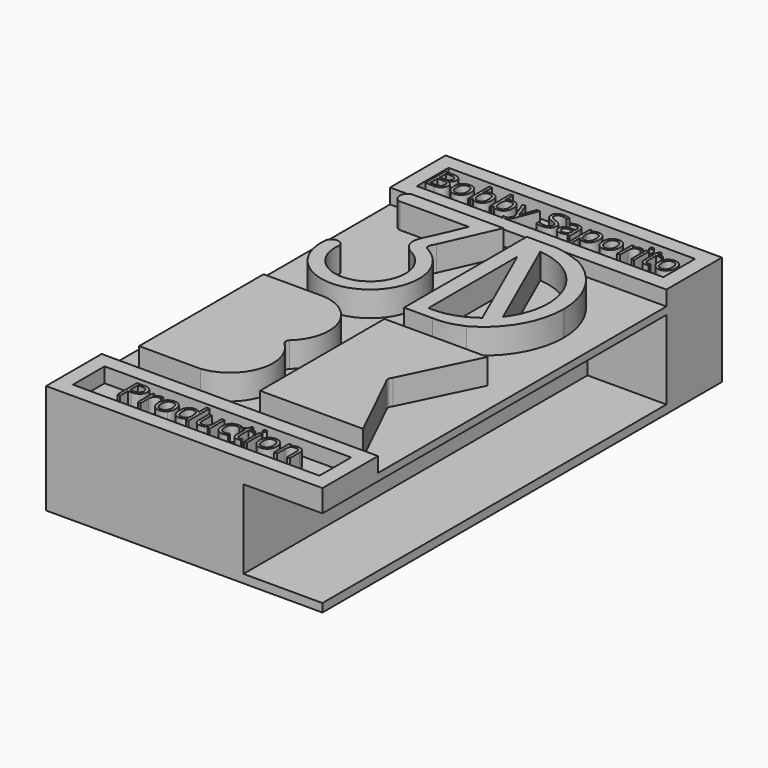
from build123d import *

# Parameters (mm, degrees)
F1_W           = 55.6107703596
F1_H           = 92.8997322917
F2_DEPTH       = 19.05
F3_DEPTH       = 5.08
F5_DEPTH       = 3
F6_DEPTH       = 3
F7_W           = 55.6107703596
F7_H           = 3.7946861994
F8_DEPTH       = 19.05
F9_W           = 55.6107703596
F9_H           = 3.7949544203
F10_DEPTH      = 19.05
F11_W          = 15.875
F11_H          = 7.9375
F11_W_2        = 15.8749995753
F12_DEPTH      = 86.5193729115
F4_TEXT_SIZE   = 6.9556654327
F13_DEPTH      = 3
F4_TEXT_SIZE_2 = 6.995924438
F14_DEPTH      = 3


# Not quite as in the source:
# - ends of sketch curves that miss each other by under 0.0002 mm in the source are joined
# - a feature names something its author has since deleted; it is built from what else it names
# - Text() gives the source's letters only with a copy of the font that has no kerning and outlines rounded to 1/6400 em; it was checked with that copy


with BuildPart() as f2:
    # F1 (on Top) → F2 (new body)
    with BuildSketch(Plane.XY):
        with Locations((-0.0001015142, 0.0001341105)):
            Rectangle(F1_W, F1_H)
    extrude(amount=-F2_DEPTH)

    # F0 (on Top) → F3 (join)
    with BuildSketch(Plane.XY):
        with BuildLine():
            Line((1.9535701722, 33.4806852043), (1.9535701722, 2.6171170175))
            Line((1.9535701722, 2.6171170175), (7.6673883013, 2.6171170175))
            add(Edge.make_bspline(
                [(13.5640528841, 3.8033656441), (12.5585792201, 3.4051600509), (10.5947152477, 2.6273956539), (8.6274422547, 2.6204880265), (7.6673883013, 2.6171170175)],
                knots=[0, 0, 0, 0, 0.5119874279, 1, 1, 1, 1], degree=3))
            ThreePointArc((13.5640528841, 3.8033656441), (19.5771167094, 9.6257290209), (21.8482203782, 17.6817168551))
            Line((21.8482203782, 17.6817168551), (21.8482203782, 18.0489011109))
            ThreePointArc((21.8482203782, 18.0489011109), (19.5771167094, 26.1048889451), (13.5640528841, 31.9272523219))
            add(Edge.make_bspline(
                [(13.5640528841, 31.9272523219), (12.0188625137, 32.4806988664), (9.5071250594, 33.3803371514), (8.1786150797, 33.4528004476), (7.6673883013, 33.4806852043)],
                knots=[0, 0, 0, 0, 0.6151878524, 1, 1, 1, 1], degree=3))
            Line((7.6673883013, 33.4806852043), (1.9535701722, 33.4806852043))
        make_face()
        with BuildLine():
            ThreePointArc((13.7255926495, 7.5781230036), (9.6198125415, 5.4448354943), (5.0269701927, 4.8843490524))
            Line((5.0269701927, 4.8843490524), (5.0269701927, 27.2558980547))
            Line((5.0269701927, 27.2558980547), (13.7255926495, 7.5781230036))
        make_face(mode=Mode.SUBTRACT)
        with BuildLine():
            ThreePointArc((6.7811124511, 30.8286115181), (17.6657420253, 23.1223286699), (16.0391214303, 9.8854082672))
            Line((16.0391214303, 9.8854082672), (6.7811124511, 30.8286115181))
        make_face(mode=Mode.SUBTRACT)
        with BuildLine():
            Line((-7.5453622267, 22.6989928633), (-2.7351737954, 33.4806852043))
            Line((-2.7351737954, 33.4806852043), (-21.1572051048, 33.4806852043))
            ThreePointArc((-21.1572051048, 33.4806852043), (-22.3890896886, 31.9530339911), (-21.1572051048, 30.425382778))
            Line((-21.1572051048, 30.425382778), (-7.2931135073, 30.425382778))
            Line((-7.2931135073, 30.425382778), (-9.4495294616, 25.3879800439))
            add(Edge.make_bspline(
                [(-9.4495294616, 25.3879800439), (-10.3302159731, 23.6726618568), (-11.8808970013, 20.6523914937), (-10.1830913379, 19.0052173822), (-9.4495294616, 18.2935316116)],
                knots=[0, 0, 0, 0, 0.5679353107, 1, 1, 1, 1], degree=3))
            ThreePointArc((-9.4495294616, 18.2935316116), (-8.744805336, 5.5966861339), (-19.1914085299, 12.8475483507))
            ThreePointArc((-19.1914085299, 12.8475483507), (-20.5873309935, 13.9352987723), (-21.9832534571, 12.8475483507))
            ThreePointArc((-21.9832534571, 12.8475483507), (-7.5716745464, 3.0830422585), (-7.6246123494, 20.4909825018))
            add(Edge.make_bspline(
                [(-7.5453622267, 22.6989928633), (-7.8757345138, 22.1285959519), (-8.4306078493, 21.1705917574), (-7.8693930702, 20.681447967), (-7.6246123494, 20.4909825018)],
                knots=[0, 0, 0, 0, 0.5706142153, 0.9583691649, 0.9583691649, 0.9583691649, 0.9583691649], degree=3))
        make_face()
        with BuildLine():
            Line((1.9535701722, -33.6182080209), (21.8482203782, -33.6182080209))
            Line((21.8482203782, -33.6182080209), (22.670282051, -33.6182080209))
            Line((22.670282051, -33.6182080209), (15.4876355082, -18.8196848612))
            add(Edge.make_bspline(
                [(15.4876355082, -18.8196848612), (15.371168109, -18.6560732739), (15.159509665, -18.3587387901), (15.1679139181, -18.0863425739), (15.171693638, -17.9638353875)],
                knots=[0, 0, 0, 0, 0.550261057, 1, 1, 1, 1], degree=3))
            add(Edge.make_bspline(
                [(15.4876355082, -17.1079859138), (15.371168109, -17.2715975011), (15.159509665, -17.5689319849), (15.1679139181, -17.8413282011), (15.171693638, -17.9638353875)],
                knots=[0, 0, 0, 0, 0.550261057, 1, 1, 1, 1], degree=3))
            Line((15.4876355082, -17.1079859138), (22.670282051, -2.3094627541))
            Line((22.670282051, -2.3094627541), (1.9535701722, -2.3094627541))
            Line((1.9535701722, -2.3094627541), (1.9535701722, -33.6182080209))
        make_face()
        with BuildLine():
            Line((-22.3890896886, -2.3094627541), (-22.3890896886, -33.6182080209))
            Line((-22.3890896886, -33.6182080209), (-10.0687015802, -33.6182080209))
            ThreePointArc((-10.0687015802, -33.6182080209), (-2.7489802993, -27.706179837), (-5.1699676551, -18.6139184516))
            add(Edge.make_bspline(
                [(-5.1699676551, -18.6139184516), (-5.2577137292, -18.4897791328), (-5.4173213156, -18.2639732804), (-5.4122223799, -18.0570156997), (-5.4099266417, -17.9638353875)],
                knots=[0, 0, 0, 0, 0.5497612996, 1, 1, 1, 1], degree=3))
            add(Edge.make_bspline(
                [(-5.1699676551, -17.3137523234), (-5.2577137292, -17.4378916422), (-5.4173213156, -17.6636974946), (-5.4122223799, -17.8706550753), (-5.4099266417, -17.9638353875)],
                knots=[0, 0, 0, 0, 0.5497612996, 1, 1, 1, 1], degree=3))
            ThreePointArc((-5.1699676551, -17.3137523234), (-2.7489802993, -8.221490938), (-10.0687015802, -2.3094627541))
            Line((-10.0687015802, -2.3094627541), (-22.3890896886, -2.3094627541))
        make_face()
    extrude(amount=F3_DEPTH)

    # F4 (on face) → F5 (join)
    with BuildSketch(Plane.XY):
        Polygon((-27.805486694, 46.4500002563), (-27.805486694, 36.2746864557), (27.8052836657, 36.2746864557), (27.8052836657, 46.4500002563), (24.8052836657, 46.4500002563), (24.8052836657, 39.2746864557), (-24.805486694, 39.2746864557), (-24.805486694, 46.4500002563), align=None)
        Polygon((-27.805486694, 50.2446864557), (-27.805486694, 46.4500002563), (-24.805486694, 46.4500002563), (-24.805486694, 47.2446864557), (24.8052836657, 47.2446864557), (24.8052836657, 46.4500002563), (27.8052836657, 46.4500002563), (27.8052836657, 50.2446864557), align=None)
    extrude(amount=F5_DEPTH)

    # F4 (on face) → F6 (join)
    with BuildSketch(Plane.XY):
        Polygon((27.8052836657, -36.2746864557), (-27.805486694, -36.2746864557), (-27.805486694, -46.4497320354), (-24.805486694, -46.4497320354), (-24.805486694, -39.2746864557), (24.8052836657, -39.2746864557), (24.8052836657, -46.4497320354), (27.8052836657, -46.4497320354), align=None)
        Polygon((-24.805486694, -46.4497320354), (-27.805486694, -46.4497320354), (-27.805486694, -50.2446864557), (27.8052836657, -50.2446864557), (27.8052836657, -46.4497320354), (24.8052836657, -46.4497320354), (24.8052836657, -47.2446864557), (-24.805486694, -47.2446864557), align=None)
        with BuildLine():
            add(Edge.make_bspline(
                [(-14.0935817981, -41.9836251579), (-14.0935817981, -42.7422457142), (-14.6111708952, -43.1505234919)],
                knots=[0, 0, 0, 1, 1, 1], degree=2))
            add(Edge.make_bspline(
                [(-15.9649915853, -40.5286914975), (-14.0935817981, -40.5286914975), (-14.0935817981, -41.9836251579)],
                knots=[0, 0, 0, 1, 1, 1], degree=2))
            Line((-15.9649915853, -40.5286914975), (-17.2603307195, -40.5286914975))
            Line((-17.2603307195, -40.5286914975), (-17.2603307195, -45.5231256783))
            Line((-17.2603307195, -45.5231256783), (-16.6798876138, -45.5231256783))
            Line((-16.6798876138, -45.5231256783), (-16.6798876138, -43.5588012697))
            Line((-16.6798876138, -43.5588012697), (-16.0917927157, -43.5588012697))
            add(Edge.make_bspline(
                [(-14.6111708952, -43.1505234919), (-15.1287599923, -43.5588012697), (-16.0917927157, -43.5588012697)],
                knots=[0, 0, 0, 1, 1, 1], degree=2))
        make_face()
        with BuildLine():
            Line((-16.1562863941, -43.0603416535), (-16.6798876138, -43.0603416535))
            Line((-16.6798876138, -43.0603416535), (-16.6798876138, -41.0315235664))
            Line((-16.6798876138, -41.0315235664), (-16.0305783769, -41.0315235664))
            add(Edge.make_bspline(
                [(-15.0194486729, -41.2736481388), (-15.3441032914, -41.0315235664), (-16.0305783769, -41.0315235664)],
                knots=[0, 0, 0, 1, 1, 1], degree=2))
            add(Edge.make_bspline(
                [(-14.6947940545, -42.0109529878), (-14.6947940545, -41.5157727111), (-15.0194486729, -41.2736481388)],
                knots=[0, 0, 0, 1, 1, 1], degree=2))
            add(Edge.make_bspline(
                [(-15.039671267, -42.8111118454), (-14.6947940545, -42.5618820373), (-14.6947940545, -42.0109529878)],
                knots=[0, 0, 0, 1, 1, 1], degree=2))
            add(Edge.make_bspline(
                [(-16.1562863941, -43.0603416535), (-15.3845484795, -43.0603416535), (-15.039671267, -42.8111118454)],
                knots=[0, 0, 0, 1, 1, 1], degree=2))
        make_face(mode=Mode.SUBTRACT)
        with BuildLine():
            add(Edge.make_bspline(
                [(-7.0462810399, -43.6473434384), (-7.0462810399, -44.5633722945), (-7.507028251, -45.077682052)],
                knots=[0, 0, 0, 1, 1, 1], degree=2))
            add(Edge.make_bspline(
                [(-7.5092144774, -42.2334015226), (-7.0462810399, -42.7564561857), (-7.0462810399, -43.6473434384)],
                knots=[0, 0, 0, 1, 1, 1], degree=2))
            add(Edge.make_bspline(
                [(-8.7570031877, -41.7103468596), (-7.9721479148, -41.7103468596), (-7.5092144774, -42.2334015226)],
                knots=[0, 0, 0, 1, 1, 1], degree=2))
            add(Edge.make_bspline(
                [(-10.0282938317, -42.2213772775), (-9.5702794036, -41.7103468596), (-8.7570031877, -41.7103468596)],
                knots=[0, 0, 0, 1, 1, 1], degree=2))
            add(Edge.make_bspline(
                [(-10.4863082597, -43.6473434384), (-10.4863082597, -42.7324076954), (-10.0282938317, -42.2213772775)],
                knots=[0, 0, 0, 1, 1, 1], degree=2))
            add(Edge.make_bspline(
                [(-10.2742443002, -44.679242293), (-10.4863082597, -44.238717676), (-10.4863082597, -43.6473434384)],
                knots=[0, 0, 0, 1, 1, 1], degree=2))
            add(Edge.make_bspline(
                [(-9.6730320438, -45.3558793597), (-10.0621803407, -45.1197669099), (-10.2742443002, -44.679242293)],
                knots=[0, 0, 0, 1, 1, 1], degree=2))
            add(Edge.make_bspline(
                [(-8.7810516779, -45.5919918095), (-9.2838837469, -45.5919918095), (-9.6730320438, -45.3558793597)],
                knots=[0, 0, 0, 1, 1, 1], degree=2))
            add(Edge.make_bspline(
                [(-7.507028251, -45.077682052), (-7.967775462, -45.5919918095), (-8.7810516779, -45.5919918095)],
                knots=[0, 0, 0, 1, 1, 1], degree=2))
        make_face()
        with BuildLine():
            add(Edge.make_bspline(
                [(-9.8982133616, -43.6473434384), (-9.8982133616, -44.3655188064), (-9.6112711484, -44.7410031884)],
                knots=[0, 0, 0, 1, 1, 1], degree=2))
            add(Edge.make_bspline(
                [(-9.6145504879, -42.5580561411), (-9.8982133616, -42.9237025043), (-9.8982133616, -43.6473434384)],
                knots=[0, 0, 0, 1, 1, 1], degree=2))
            add(Edge.make_bspline(
                [(-8.7744929988, -42.1924097779), (-9.3308876142, -42.1924097779), (-9.6145504879, -42.5580561411)],
                knots=[0, 0, 0, 1, 1, 1], degree=2))
            add(Edge.make_bspline(
                [(-7.9218647079, -42.5629751505), (-8.210446591, -42.1924097779), (-8.7744929988, -42.1924097779)],
                knots=[0, 0, 0, 1, 1, 1], degree=2))
            add(Edge.make_bspline(
                [(-7.6332828248, -43.6473434384), (-7.6332828248, -42.933540523), (-7.9218647079, -42.5629751505)],
                knots=[0, 0, 0, 1, 1, 1], degree=2))
            add(Edge.make_bspline(
                [(-7.9218647079, -44.7426428582), (-7.6332828248, -44.368798146), (-7.6332828248, -43.6473434384)],
                knots=[0, 0, 0, 1, 1, 1], degree=2))
            add(Edge.make_bspline(
                [(-8.7679343196, -45.1164875703), (-8.210446591, -45.1164875703), (-7.9218647079, -44.7426428582)],
                knots=[0, 0, 0, 1, 1, 1], degree=2))
            add(Edge.make_bspline(
                [(-9.6112711484, -44.7410031884), (-9.3243289351, -45.1164875703), (-8.7679343196, -45.1164875703)],
                knots=[0, 0, 0, 1, 1, 1], degree=2))
        make_face(mode=Mode.SUBTRACT)
        with BuildLine():
            Line((-3.5341083494, -45.0213867225), (-3.50350118, -45.0213867225))
            Line((-3.50350118, -45.0213867225), (-3.4280763696, -45.5231256783))
            Line((-3.4280763696, -45.5231256783), (-2.966782602, -45.5231256783))
            Line((-2.966782602, -45.5231256783), (-2.966782602, -40.2073162186))
            Line((-2.966782602, -40.2073162186), (-3.5341083494, -40.2073162186))
            Line((-3.5341083494, -40.2073162186), (-3.5341083494, -41.7311160102))
            Line((-3.5341083494, -41.7311160102), (-3.5198978779, -41.9945562899))
            Line((-3.5198978779, -41.9945562899), (-3.4958493876, -42.2645552486))
            Line((-3.4958493876, -42.2645552486), (-3.5406670286, -42.2645552486))
            add(Edge.make_bspline(
                [(-4.7092050324, -41.7103468596), (-3.9473051365, -41.7103468596), (-3.5406670286, -42.2645552486)],
                knots=[0, 0, 0, 1, 1, 1], degree=2))
            add(Edge.make_bspline(
                [(-5.8504152063, -42.2230169473), (-5.4404977588, -41.7103468596), (-4.7092050324, -41.7103468596)],
                knots=[0, 0, 0, 1, 1, 1], degree=2))
            add(Edge.make_bspline(
                [(-6.2603326539, -43.6615539099), (-6.2603326539, -42.735687035), (-5.8504152063, -42.2230169473)],
                knots=[0, 0, 0, 1, 1, 1], degree=2))
            add(Edge.make_bspline(
                [(-5.8520548761, -45.0897062971), (-6.2603326539, -44.5874207847), (-6.2603326539, -43.6615539099)],
                knots=[0, 0, 0, 1, 1, 1], degree=2))
            add(Edge.make_bspline(
                [(-4.7092050324, -45.5919918095), (-5.4437770984, -45.5919918095), (-5.8520548761, -45.0897062971)],
                knots=[0, 0, 0, 1, 1, 1], degree=2))
            add(Edge.make_bspline(
                [(-3.5341083494, -45.0213867225), (-3.9265359859, -45.5919918095), (-4.7092050324, -45.5919918095)],
                knots=[0, 0, 0, 1, 1, 1], degree=2))
        make_face()
        with BuildLine():
            add(Edge.make_bspline(
                [(-4.6370595616, -45.1164875703), (-4.0566164559, -45.1164875703), (-3.7953624026, -44.8005778574)],
                knots=[0, 0, 0, 1, 1, 1], degree=2))
            add(Edge.make_bspline(
                [(-5.4093440328, -44.7508412071), (-5.1464503097, -45.1164875703), (-4.6370595616, -45.1164875703)],
                knots=[0, 0, 0, 1, 1, 1], degree=2))
            add(Edge.make_bspline(
                [(-5.6722377558, -43.668112589), (-5.6722377558, -44.3851948439), (-5.4093440328, -44.7508412071)],
                knots=[0, 0, 0, 1, 1, 1], degree=2))
            add(Edge.make_bspline(
                [(-5.407704363, -42.5733597258), (-5.6722377558, -42.9608683529), (-5.6722377558, -43.668112589)],
                knots=[0, 0, 0, 1, 1, 1], degree=2))
            add(Edge.make_bspline(
                [(-4.6436182408, -42.1858510987), (-5.1431709702, -42.1858510987), (-5.407704363, -42.5733597258)],
                knots=[0, 0, 0, 1, 1, 1], degree=2))
            add(Edge.make_bspline(
                [(-3.7986417422, -42.5258093019), (-4.063175135, -42.1858510987), (-4.6436182408, -42.1858510987)],
                knots=[0, 0, 0, 1, 1, 1], degree=2))
            add(Edge.make_bspline(
                [(-3.5341083494, -43.6615539099), (-3.5341083494, -42.865767505), (-3.7986417422, -42.5258093019)],
                knots=[0, 0, 0, 1, 1, 1], degree=2))
            Line((-3.5341083494, -43.6615539099), (-3.5341083494, -43.780703248))
            add(Edge.make_bspline(
                [(-3.7953624026, -44.8005778574), (-3.5341083494, -44.4846681445), (-3.5341083494, -43.780703248)],
                knots=[0, 0, 0, 1, 1, 1], degree=2))
        make_face(mode=Mode.SUBTRACT)
        with BuildLine():
            add(Edge.make_bspline(
                [(7.069089627, -45.1230462495), (7.2199392477, -45.1230462495), (7.3598577364, -45.1011839856)],
                knots=[0, 0, 0, 1, 1, 1], degree=2))
            add(Edge.make_bspline(
                [(6.62856501, -44.942136016), (6.7892526495, -45.1230462495), (7.069089627, -45.1230462495)],
                knots=[0, 0, 0, 1, 1, 1], degree=2))
            add(Edge.make_bspline(
                [(6.4678773706, -44.4234538057), (6.4678773706, -44.7612257825), (6.62856501, -44.942136016)],
                knots=[0, 0, 0, 1, 1, 1], degree=2))
            Line((6.4678773706, -44.4234538057), (6.4678773706, -42.2197376077))
            Line((6.4678773706, -42.2197376077), (7.5544318849, -42.2197376077))
            Line((7.5544318849, -42.2197376077), (7.5544318849, -41.7792129908))
            Line((7.5544318849, -41.7792129908), (6.4678773706, -41.7792129908))
            Line((6.4678773706, -41.7792129908), (6.4678773706, -40.9112811152))
            Line((6.4678773706, -40.9112811152), (6.1399434126, -40.9112811152))
            Line((6.1399434126, -40.9112811152), (5.9016447364, -41.7103468596))
            Line((5.9016447364, -41.7103468596), (5.3649261584, -41.9464593094))
            Line((5.3649261584, -41.9464593094), (5.3649261584, -42.2197376077))
            Line((5.3649261584, -42.2197376077), (5.9016447364, -42.2197376077))
            Line((5.9016447364, -42.2197376077), (5.9016447364, -44.447502296))
            add(Edge.make_bspline(
                [(6.9871061375, -45.5919918095), (5.9016447364, -45.5919918095), (5.9016447364, -44.447502296)],
                knots=[0, 0, 0, 1, 1, 1], degree=2))
            add(Edge.make_bspline(
                [(7.3106676427, -45.5624777533), (7.131397079, -45.5919918095), (6.9871061375, -45.5919918095)],
                knots=[0, 0, 0, 1, 1, 1], degree=2))
            add(Edge.make_bspline(
                [(7.5817597147, -45.4892391693), (7.4899382065, -45.532963697), (7.3106676427, -45.5624777533)],
                knots=[0, 0, 0, 1, 1, 1], degree=2))
            Line((7.5817597147, -45.4892391693), (7.5817597147, -45.0552732315))
            add(Edge.make_bspline(
                [(7.3598577364, -45.1011839856), (7.4997762252, -45.0793217218), (7.5817597147, -45.0552732315)],
                knots=[0, 0, 0, 1, 1, 1], degree=2))
        make_face()
        with BuildLine():
            Line((-1.2309188508, -44.2081105066), (-1.2309188508, -41.7792129908))
            Line((-1.2309188508, -41.7792129908), (-1.8048032774, -41.7792129908))
            Line((-1.8048032774, -41.7792129908), (-1.8048032774, -44.2288796573))
            add(Edge.make_bspline(
                [(-1.4653916308, -45.267337191), (-1.8048032774, -44.9426825726), (-1.8048032774, -44.2288796573)],
                knots=[0, 0, 0, 1, 1, 1], degree=2))
            add(Edge.make_bspline(
                [(-0.4427842384, -45.5919918095), (-1.1259799843, -45.5919918095), (-1.4653916308, -45.267337191)],
                knots=[0, 0, 0, 1, 1, 1], degree=2))
            add(Edge.make_bspline(
                [(0.2633668846, -45.444968085), (-0.0459841491, -45.5919918095), (-0.4427842384, -45.5919918095)],
                knots=[0, 0, 0, 1, 1, 1], degree=2))
            add(Edge.make_bspline(
                [(0.7465229161, -45.0213867225), (0.5727179184, -45.2979443605), (0.2633668846, -45.444968085)],
                knots=[0, 0, 0, 1, 1, 1], degree=2))
            Line((0.7465229161, -45.0213867225), (0.7771300855, -45.0213867225))
            Line((0.7771300855, -45.0213867225), (0.859113575, -45.5231256783))
            Line((0.859113575, -45.5231256783), (1.3269660218, -45.5231256783))
            Line((1.3269660218, -45.5231256783), (1.3269660218, -41.7792129908))
            Line((1.3269660218, -41.7792129908), (0.7596402744, -41.7792129908))
            Line((0.7596402744, -41.7792129908), (0.7596402744, -43.746816739))
            add(Edge.make_bspline(
                [(0.4885482025, -44.7956588481), (0.7596402744, -44.4748301258), (0.7596402744, -43.746816739)],
                knots=[0, 0, 0, 1, 1, 1], degree=2))
            add(Edge.make_bspline(
                [(-0.3706387676, -45.1164875703), (0.2174561305, -45.1164875703), (0.4885482025, -44.7956588481)],
                knots=[0, 0, 0, 1, 1, 1], degree=2))
            add(Edge.make_bspline(
                [(-1.0226807875, -44.8913062525), (-0.8144427241, -45.1164875703), (-0.3706387676, -45.1164875703)],
                knots=[0, 0, 0, 1, 1, 1], degree=2))
            add(Edge.make_bspline(
                [(-1.2309188508, -44.2081105066), (-1.2309188508, -44.6661249346), (-1.0226807875, -44.8913062525)],
                knots=[0, 0, 0, 1, 1, 1], degree=2))
        make_face()
    extrude(amount=F6_DEPTH)

    # F7 (on face) → F8 (join, through all)
    with BuildSketch(Plane(origin=(0, 0, 0), x_dir=(1, 0, 0), z_dir=(0, 0, -1))):
        with Locations((-0.0001015142, -48.347343356)):
            Rectangle(F7_W, F7_H)
    extrude(amount=F8_DEPTH)

    # F9 (on face) → F10 (join, through all)
    with BuildSketch(Plane(origin=(0, 0, 0), x_dir=(1, 0, 0), z_dir=(0, 0, -1))):
        with Locations((-0.0001015142, 48.3472092456)):
            Rectangle(F9_W, F9_H)
    extrude(amount=F10_DEPTH)

    # F11 (on face) → F12 (cut, through all)
    with BuildSketch(Plane.XZ.offset(50.2446864557)):
        with Locations((19.8677840903, -5.4532486349)):
            Rectangle(F11_W, F11_H)
        with Locations((19.867783878, -13.3907486349)):
            Rectangle(F11_W_2, F11_H)
    extrude(amount=-F12_DEPTH, mode=Mode.SUBTRACT)

    # F4 (on face) → F13 (join)
    with BuildSketch(Plane.XY):
        with Locations((-25.1435358077, 40.9764871001)):
            Text('Bobby Saporito', F4_TEXT_SIZE, font='Open Sans', text_align=(TextAlign.LEFT, TextAlign.BOTTOM))
    extrude(amount=F13_DEPTH)

    # F4 (on face) → F14 (join)
    with BuildSketch(Plane.XY):
        with Locations((-17.946805805, -45.5231256783)):
            Text('Production', F4_TEXT_SIZE_2, font='Open Sans', text_align=(TextAlign.LEFT, TextAlign.BOTTOM))
    extrude(amount=F14_DEPTH)


solid = f2.part
